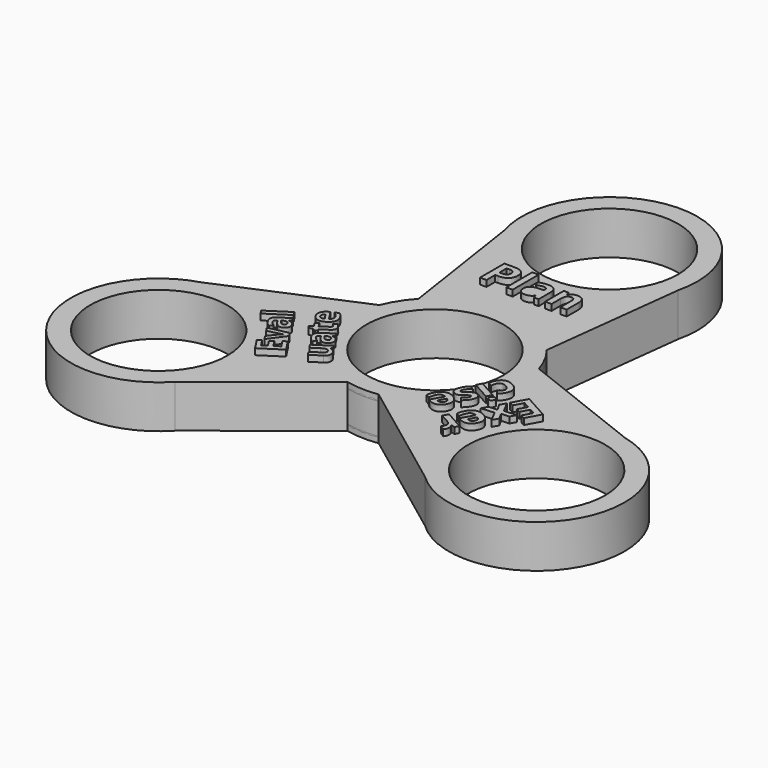
from build123d import *

# Parameters (mm, degrees)
F0_R           = 11.15
F1_DEPTH       = 7
F2_R           = 0.9999
F3_TEXT_SIZE   = 6.9444444444
F4_DEPTH       = 8
F5_TEXT_SIZE   = 5.5555555556
F6_DEPTH       = 8
F7_TEXT_SIZE   = 6.4113204207
F7_TEXT_SIZE_2 = 6.25
F8_DEPTH       = 8
F9_DEPTH       = 8
F10_DEPTH      = 7


# Not quite as in the source:
# - a fillet or chamfer is up to 0.001 mm smaller than in the source, because OpenCascade refuses the exact size
# - Text() gives the source's letters only with a copy of the font that has no kerning and outlines rounded to 1/6400 em; it was checked with that copy


with BuildPart() as f1:
    # F0 (on Top) → F1 (new body)
    with BuildSketch(Plane.XY):
        with BuildLine():
            Line((-20.2812175918, -27.497935086), (-3.1674683079, -13.8422232506))
            ThreePointArc((-3.1674683079, -13.8422232506), (-0.5500071761, -14.1893443156), (2.0864701614, -14.0458763438))
            Line((2.0864701614, -14.0458763438), (20.8507180686, -28.075449868))
            ThreePointArc((20.8507180686, -28.075449868), (43.3258545673, -24.5459153486), (33.954519132, -3.8150821112))
            Line((33.954519132, -3.8150821112), (13.5714511338, 4.178003605))
            ThreePointArc((13.5714511338, 4.178003605), (12.5633362284, 6.618351971), (11.1208506514, 8.8298743359))
            Line((11.1208506514, 8.8298743359), (13.8886937741, 32.0949764686))
            ThreePointArc((13.8886937741, 32.0949764686), (-0.4055410326, 49.7942483703), (-13.6733015402, 31.3130171971))
            Line((-13.6733015402, 31.3130171971), (-10.4039828259, 9.6642196456))
            ThreePointArc((-10.4039828259, 9.6642196456), (-12.0133290523, 7.5709923446), (-13.2073208129, 5.2160020079))
            Line((-13.2073208129, 5.2160020079), (-34.7394118427, -4.0195266005))
            ThreePointArc((-34.7394118427, -4.0195266005), (-42.9203135347, -25.2483330217), (-20.2812175918, -27.497935086))
        make_face()
        with Locations((-30.7439018343, -17.75)):
            Circle(F0_R, mode=Mode.SUBTRACT)
        with Locations((30.7439018343, -17.75)):
            Circle(F0_R, mode=Mode.SUBTRACT)
        Circle(F0_R, mode=Mode.SUBTRACT)
        with Locations((0, 35.5)):
            Circle(F0_R, mode=Mode.SUBTRACT)
    extrude(amount=F1_DEPTH)

    # F2 (radius 1 in the source; OpenCascade refuses exactly that, so slightly less here)
    f2_edges = [f1.edges().sort_by_distance(p)[0] for p in [
        (-0.405541, 49.794248, 7),
        (-0.405541, 49.794248, 0),
        (-10.403983, 9.66422, 3.5),
        (-12.038642, 20.488618, 7),
        (-12.038642, 20.488618, 0),
        (-23.973366, 0.598238, 0),
        (-12.013329, 7.570992, 0),
        (-12.013329, 7.570992, 7),
        (-23.973366, 0.598238, 7),
        (-42.920314, -25.248333, 0),
        (-42.920314, -25.248333, 7),
        (-11.724343, -20.670079, 0),
        (-11.724343, -20.670079, 7),
        (-0.550007, -14.189344, 7),
        (-0.550007, -14.189344, 0),
        (11.468594, -21.060663, 7),
        (11.468594, -21.060663, 0),
        (43.325855, -24.545915, 7),
        (43.325855, -24.545915, 0),
        (23.762985, 0.181461, 7),
        (23.762985, 0.181461, 0),
        (12.563336, 6.618352, 0),
        (12.563336, 6.618352, 7),
        (12.504772, 20.462425, 7),
        (12.504772, 20.462425, 0),
    ]]
    fillet(f2_edges, radius=F2_R)

    # F5 (on Top) → F6 (join)
    with BuildSketch(Plane.XY):
        with Locations(Location((-13.3324329355, -13.6861392512), (0, 0, 122.9187655143))):
            Text('Eval', F5_TEXT_SIZE, font='Open Sans', font_style=FontStyle.BOLD, text_align=(TextAlign.LEFT, TextAlign.BOTTOM))
        with Locations(Location((-7.7839250633, -11.3445207073), (0, 0, 123.1349212679))):
            Text('uate', F5_TEXT_SIZE, font='Open Sans', font_style=FontStyle.BOLD, text_align=(TextAlign.LEFT, TextAlign.BOTTOM))
    extrude(amount=F6_DEPTH)

    # F7 (on Top) → F8 (join)
    with BuildSketch(Plane.XY):
        with Locations(Location((19.2888936952, -4.0762271619), (0, 0, -118.9612627301))):
            Text('Exer', F7_TEXT_SIZE, font='Open Sans', font_style=FontStyle.BOLD, text_align=(TextAlign.LEFT, TextAlign.BOTTOM))
        with Locations(Location((13.5008720234, -1.7320023349), (0, 0, -118.8492104109))):
            Text('cise', F7_TEXT_SIZE_2, font='Open Sans', font_style=FontStyle.BOLD, text_align=(TextAlign.LEFT, TextAlign.BOTTOM))
    extrude(amount=F8_DEPTH)

    # F7 (on Top) → F9 (join)
    with BuildSketch(Plane.XY):
        with Locations(Location((19.2888936952, -4.0762271619), (0, 0, -118.9612627301))):
            Text('Exer', F7_TEXT_SIZE, font='Open Sans', font_style=FontStyle.BOLD, text_align=(TextAlign.LEFT, TextAlign.BOTTOM))
        with Locations(Location((13.5008720234, -1.7320023349), (0, 0, -118.8492104109))):
            Text('cise', F7_TEXT_SIZE_2, font='Open Sans', font_style=FontStyle.BOLD, text_align=(TextAlign.LEFT, TextAlign.BOTTOM))
    extrude(amount=F9_DEPTH)


with BuildPart() as f4:
    # F3 (on Top) → F4 (new body)
    with BuildSketch(Plane.XY):
        with Locations((-7.3669040576, 17.5978779296)):
            Text('Plan', F3_TEXT_SIZE, font='Open Sans', font_style=FontStyle.BOLD, text_align=(TextAlign.LEFT, TextAlign.BOTTOM))
        with BuildLine():
            Line((1.7585299702, 19.0421053602), (1.7585299702, 19.3546053602))
            Line((1.7585299702, 19.3546053602), (1.3581393452, 19.3404994574))
            add(Edge.make_bspline(
                [(1.3581393452, 19.3404994574), (0.9067504563, 19.3274786241), (0.6864813591, 19.1782815754)],
                knots=[0, 0, 0, 1, 1, 1], degree=2))
            add(Edge.make_bspline(
                [(0.6864813591, 19.1782815754), (0.4662122619, 19.0290845268), (0.4662122619, 18.7241800129)],
                knots=[0, 0, 0, 1, 1, 1], degree=2))
            add(Edge.make_bspline(
                [(0.4662122619, 18.7241800129), (0.4662122619, 18.2858119574), (0.9675143452, 18.2858119574)],
                knots=[0, 0, 0, 1, 1, 1], degree=2))
            add(Edge.make_bspline(
                [(0.9675143452, 18.2858119574), (1.3277574008, 18.2858119574), (1.5431436855, 18.4930602213)],
                knots=[0, 0, 0, 1, 1, 1], degree=2))
            add(Edge.make_bspline(
                [(1.5431436855, 18.4930602213), (1.7585299702, 18.7003084852), (1.7585299702, 19.0421053602)],
                knots=[0, 0, 0, 1, 1, 1], degree=2))
        make_face()
    extrude(amount=F4_DEPTH)


with BuildPart() as f10:
    # F0 (on Top) → F10 (new body)
    with BuildSketch(Plane.XY):
        with BuildLine():
            Line((-20.2812175918, -27.497935086), (-3.1674683079, -13.8422232506))
            ThreePointArc((-3.1674683079, -13.8422232506), (-0.5500071761, -14.1893443156), (2.0864701614, -14.0458763438))
            Line((2.0864701614, -14.0458763438), (20.8507180686, -28.075449868))
            ThreePointArc((20.8507180686, -28.075449868), (43.3258545673, -24.5459153486), (33.954519132, -3.8150821112))
            Line((33.954519132, -3.8150821112), (13.5714511338, 4.178003605))
            ThreePointArc((13.5714511338, 4.178003605), (12.5633362284, 6.618351971), (11.1208506514, 8.8298743359))
            Line((11.1208506514, 8.8298743359), (13.8886937741, 32.0949764686))
            ThreePointArc((13.8886937741, 32.0949764686), (-0.4055410326, 49.7942483703), (-13.6733015402, 31.3130171971))
            Line((-13.6733015402, 31.3130171971), (-10.4039828259, 9.6642196456))
            ThreePointArc((-10.4039828259, 9.6642196456), (-12.0133290523, 7.5709923446), (-13.2073208129, 5.2160020079))
            Line((-13.2073208129, 5.2160020079), (-34.7394118427, -4.0195266005))
            ThreePointArc((-34.7394118427, -4.0195266005), (-42.9203135347, -25.2483330217), (-20.2812175918, -27.497935086))
        make_face()
        with Locations((-30.7439018343, -17.75)):
            Circle(F0_R, mode=Mode.SUBTRACT)
        with Locations((30.7439018343, -17.75)):
            Circle(F0_R, mode=Mode.SUBTRACT)
        Circle(F0_R, mode=Mode.SUBTRACT)
        with Locations((0, 35.5)):
            Circle(F0_R, mode=Mode.SUBTRACT)
    extrude(amount=F10_DEPTH)


solid = Compound([f1.part, f4.part, f10.part])
